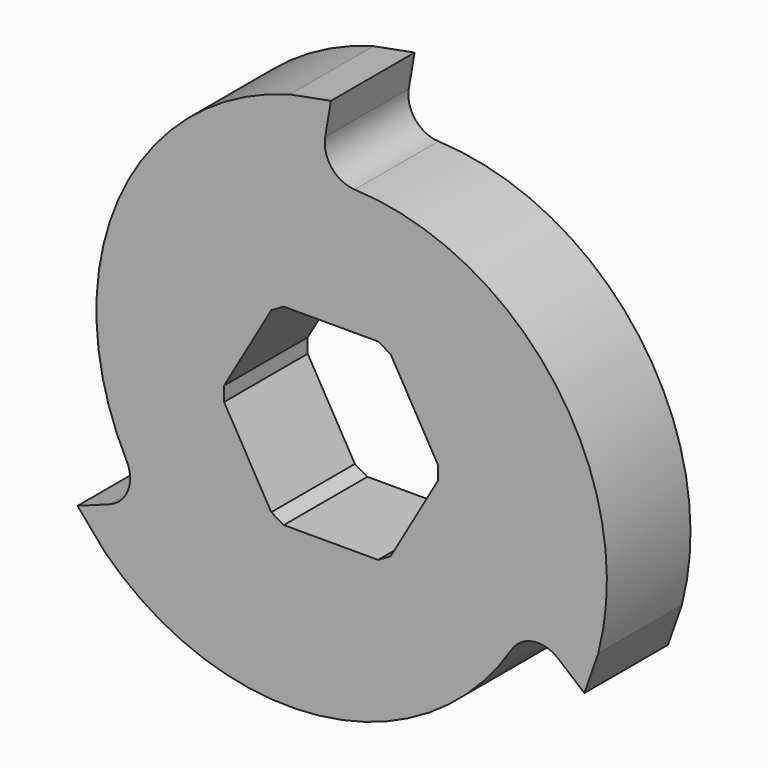
from build123d import *

# Parameters (mm, degrees)
F1_DEPTH = 50


# Not quite as in the source:
# - ends of sketch curves that miss each other by under 0.0002 mm in the source are joined


with BuildPart() as f1:
    # F0 (on Front) → F1 (new body)
    with BuildSketch(Plane.XZ):
        with BuildLine():
            Line((-719.030741, 535.802017), (-716.260339, 551.935195))
            Line((-716.260339, 551.935195), (-735.912365, 548.229318))
            ThreePointArc((-735.912365, 548.229318), (-818.0414227516, 477.1771162339), (-814.0615494377, 368.65173577))
            ThreePointArc((-814.0615494377, 368.65173577), (-813.3377138775, 356.2962207865), (-822.1469540915, 347.602546248))
            Line((-822.1469540915, 347.602546248), (-837.503896, 341.935195))
            Line((-837.503896, 341.935195), (-824.468499, 326.76898))
            ThreePointArc((-824.468499, 326.76898), (-721.8709589722, 291.1692315288), (-629.8751597113, 348.8785918176))
            ThreePointArc((-629.8751597113, 348.8785918176), (-619.5368877345, 355.6832101227), (-607.6033241523, 352.4010218168))
            Line((-607.6033241523, 352.4010218168), (-595.016783, 341.935195))
            Line((-595.016783, 341.935195), (-588.400154, 360.807287))
            ThreePointArc((-588.400154, 360.807287), (-608.868637199, 467.4592376194), (-704.8443090013, 518.2752569674))
            ThreePointArc((-704.8443090013, 518.2752569674), (-715.9064175677, 523.8261534239), (-719.030741, 535.802017))
        make_face()
        Polygon((-767.376564, 415.399297), (-744.818452, 454.471094), (-738.818452, 457.935195), (-693.702227, 457.935195), (-687.702227, 454.471094), (-665.144115, 415.399297), (-665.144115, 408.471094), (-687.702227, 369.399297), (-693.702227, 365.935195), (-738.818452, 365.935195), (-744.818452, 369.399297), (-767.376564, 408.471094), align=None, mode=Mode.SUBTRACT)
    extrude(amount=F1_DEPTH)


solid = f1.part
